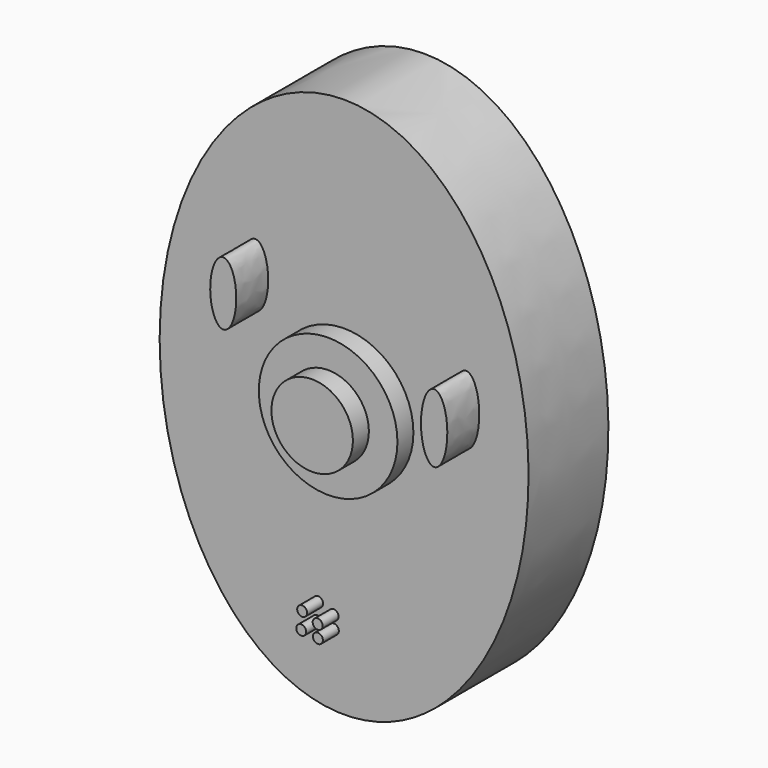
from build123d import *

# Parameters (mm, degrees)
F1_DEPTH  = 25
F3_DEPTH  = 10
F4_R      = 10.2061926116
F5_DEPTH  = 10
F6_R      = 17.3624209795
F7_DEPTH  = 5
F25_R     = 1.25
F26_DEPTH = 5
F28_DEPTH = 10


# Not quite as in the source:
# - the program builds the solid bodies; features that only make, move or delete a surface that nothing else refers to are left out


with BuildPart() as f1:
    # F0 (on Front) → F1 (new body)
    with BuildSketch(Plane.XZ):
        with BuildLine():
            add(Edge.make_bspline(
                [(0, 67.817941308), (-80.0343626638, 67.817941308), (-40.0171813319, -33.908970654), (0, -135.635882616), (40.0171813319, -33.908970654), (80.0343626638, 67.817941308), (0, 67.817941308)],
                knots=[0, 0, 0, 2.0943951024, 2.0943951024, 4.1887902048, 4.1887902048, 6.2831853072, 6.2831853072, 6.2831853072], degree=2, weights=[1, 0.5, 1, 0.5, 1, 0.5, 1]))
        make_face()
    extrude(amount=F1_DEPTH)

    # F2 (on face) → F3 (join)
    with BuildSketch(Plane.XZ.offset(25)):
        with BuildLine():
            add(Edge.make_bspline(
                [(-22.274941206, 29.8401806504), (-27.9245384405, 29.8401806504), (-25.0997398233, 17.910759896), (-22.274941206, 5.9813391417), (-19.4501425887, 17.910759896), (-16.6253439714, 29.8401806504), (-22.274941206, 29.8401806504)],
                knots=[0, 0, 0, 2.0943951024, 2.0943951024, 4.1887902048, 4.1887902048, 6.2831853072, 6.2831853072, 6.2831853072], degree=2, weights=[1, 0.5, 1, 0.5, 1, 0.5, 1]))
        make_face()
    extrude(amount=F3_DEPTH)

    # F4 (on face) → F5 (join)
    with BuildSketch(Plane.XZ.offset(25)):
        Circle(F4_R)
    extrude(amount=F5_DEPTH)

    # F6 (on face) → F7 (join)
    with BuildSketch(Plane.XZ.offset(25)):
        Circle(F6_R)
    extrude(amount=F7_DEPTH)

    # F25 (on face) → F26 (join)
    with BuildSketch(Plane.XZ.offset(25)):
        with Locations((-6.5004567707, -45.0633225443)):
            Circle(F25_R)
        with Locations((-2.6214996293, -46.6608458069)):
            Circle(F25_R)
        with Locations((-6.7332892665, -49.3229854894)):
            Circle(F25_R)
        with Locations((-2.5671826191, -49.8007137575)):
            Circle(F25_R)
    extrude(amount=F26_DEPTH)

    # F27 (on face) → F28 (join)
    with BuildSketch(Plane.XZ.offset(25)):
        with BuildLine():
            add(Edge.make_bspline(
                [(30.5588506162, 0.7911883295), (36.2714713272, 0.7911883295), (33.4151609717, 13.6598404497), (30.5588506162, 26.5284925699), (27.7025402607, 13.6598404497), (24.8462299052, 0.7911883295), (30.5588506162, 0.7911883295)],
                knots=[0, 0, 0, 2.0943951024, 2.0943951024, 4.1887902048, 4.1887902048, 6.2831853072, 6.2831853072, 6.2831853072], degree=2, weights=[1, 0.5, 1, 0.5, 1, 0.5, 1]))
        make_face()
    extrude(amount=F28_DEPTH)


solid = f1.part
